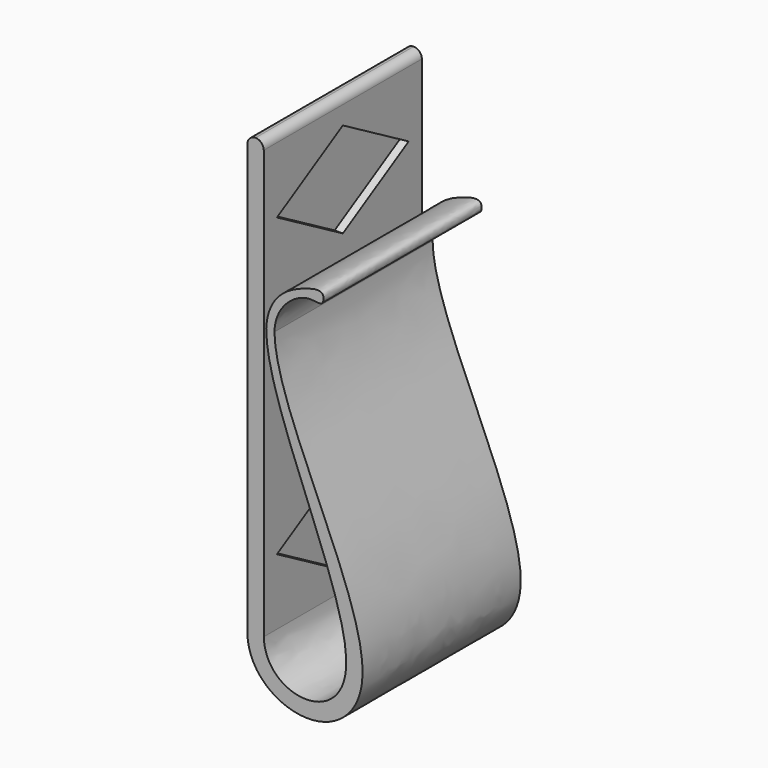
from build123d import *

# Parameters (mm, degrees)
F1_DEPTH = 24
F2_R     = 0.99999
F4_DEPTH = 1


# Not quite as in the source:
# - a fillet or chamfer is up to 0.001 mm smaller than in the source, because OpenCascade refuses the exact size


with BuildPart() as f1:
    # F0 (on Front) → F1 (new body)
    with BuildSketch(Plane.XZ):
        with BuildLine():
            Line((0, 60), (0, 6.9862387707))
            add(Edge.make_bspline(
                [(3.3, 40), (3.3994593126, 31.673934298), (19.7718344048, 7.1227607211), (7.6936961489, -2.498282177), (0, 2.5259271248), (0, 6.9862387707)],
                knots=[0, 0, 0, 0, 0.4836093037, 0.7377542004, 1, 1, 1, 1], degree=3))
            add(Edge.make_bspline(
                [(3.3, 40), (3.3385955543, 42.8341147329), (6.8505910401, 45.6295855338), (9.2446222249, 44.4214397924), (9.3793347208, 46.4252407174), (6.598029656, 45.9383519209), (2.4614556728, 43.9478391097), (2.3, 40)],
                knots=[0, 0, 0, 0, 0.2764645571, 0.4269586312, 0.5376912217, 0.6956411188, 1, 1, 1, 1], degree=3))
            add(Edge.make_bspline(
                [(2.3, 40), (2.3056045868, 31.6193630301), (17.0420838494, 6.9963103508), (7.0436122464, 0.330073677), (2.1147195613, 3.7848248686), (2, 6.9862387707)],
                knots=[0, 0, 0, 0, 0.5244829522, 0.7622414761, 1, 1, 1, 1], degree=3))
            Line((2, 6.9862387707), (2, 60))
            Line((2, 60), (0, 60))
        make_face()
    extrude(amount=F1_DEPTH)

    # F2 (radius 1 in the source; OpenCascade refuses exactly that, so slightly less here)
    f2_edges = [f1.edges().sort_by_distance(p)[0] for p in [
        (2, -12, 60),
        (0, -12, 60),
    ]]
    fillet(f2_edges, radius=F2_R)


with BuildPart() as f4:
    # F3 (on face) → F4 (new body)
    with BuildSketch(Plane.YZ.offset(2)):
        Polygon((-12, 56.7735026919), (-22, 51), (-12, 45.2264973081), (-2, 51), align=None)
    extrude(amount=-F4_DEPTH)


with BuildPart() as f1_1:
    add(f1.part)

    # F5: cut F4
    add(f4.part, mode=Mode.SUBTRACT)


with BuildPart() as f4_1:
    # F6: moved
    add(f4.part.moved(Location((0, 0, -36))))


with BuildPart() as f1_2:
    add(f1_1.part)

    # F7: cut F4
    add(f4_1.part, mode=Mode.SUBTRACT)


solid = f1_2.part
